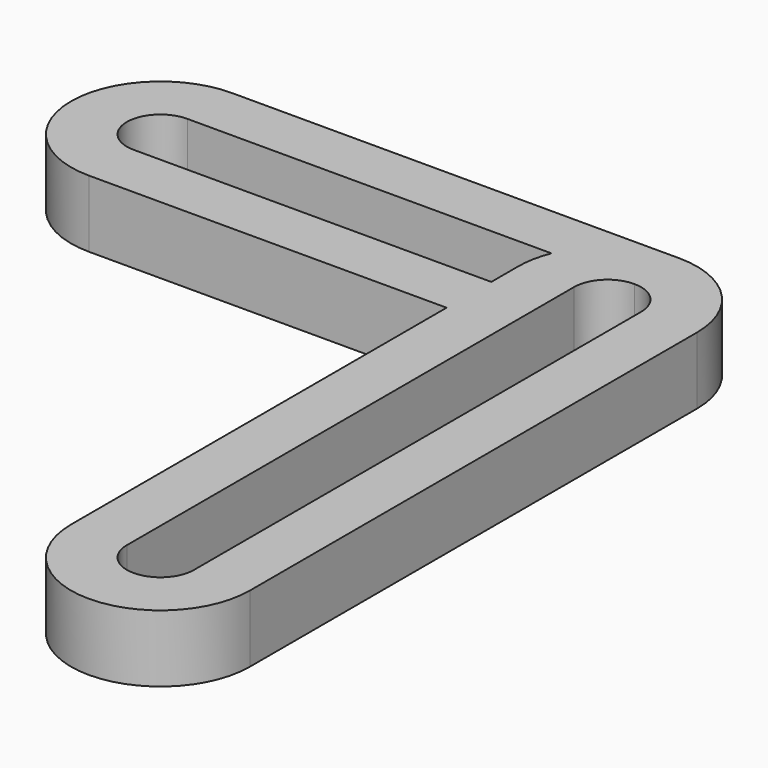
from build123d import *

# Parameters (mm, degrees)
F0_W     = 10
F0_H     = 10
F1_DEPTH = 12


# Not quite as in the source:
# - ends of sketch curves that miss each other by under 0.0002 mm in the source are joined


with BuildPart() as f1:
    # F0 (on Top) → F1 (new body)
    with BuildSketch(Plane.XY):
        with BuildLine():
            ThreePointArc((49.3437788486, 31.9918581452), (44.6574873088, 43.3055665732), (33.3437788486, 47.9918580353))
            ThreePointArc((33.3437788486, 47.9918580353), (24.3995068895, 45.2583572735), (18.51138183, 37.9918580353))
            Line((18.51138183, 37.9918580353), (33.3437788486, 37.9918580353))
            ThreePointArc((33.3437788486, 37.9918580353), (37.5864194969, 36.2344987613), (39.3437788486, 31.9918581452))
            Line((39.3437788486, 31.9918581452), (39.3437788486, 17.1594610611))
            ThreePointArc((39.3437788486, 17.1594610611), (46.6102780408, 23.0475861709), (49.3437788486, 31.9918581452))
        make_face()
        with BuildLine():
            Line((49.3437788486, -68.0081418548), (49.3437788486, 31.9918581452))
            ThreePointArc((49.3437788486, 31.9918581452), (46.6102780408, 23.0475861709), (39.3437788486, 17.1594610611))
            Line((39.3437788486, 17.1594610611), (39.3437788486, -68.0081418548))
            ThreePointArc((39.3437788486, -68.0081418548), (33.3437788486, -74.0081418548), (27.3437788486, -68.0081418548))
            Line((27.3437788486, -68.0081418548), (27.3437788486, 15.9918580353))
            Line((27.3437788486, 15.9918580353), (17.3437788486, 15.9918580353))
            Line((17.3437788486, 15.9918580353), (17.3437788486, -68.0081418548))
            ThreePointArc((17.3437788486, -68.0081418548), (33.3437788486, -84.0081418548), (49.3437788486, -68.0081418548))
        make_face()
        with BuildLine():
            Line((33.3437788486, 37.9918580353), (18.51138183, 37.9918580353))
            ThreePointArc((18.51138183, 37.9918580353), (17.6383919973, 35.0481342863), (17.3437788486, 31.9918581452))
            Line((17.3437788486, 31.9918581452), (17.3437788486, 25.9918580353))
            Line((17.3437788486, 25.9918580353), (27.3437788486, 25.9918580353))
            Line((27.3437788486, 25.9918580353), (27.3437788486, 31.9918581452))
            ThreePointArc((27.3437788486, 31.9918581452), (29.1011381615, 36.2344988323), (33.3437788486, 37.9918580353))
        make_face()
        with Locations((22.3437788486, 20.9918580353)):
            Rectangle(F0_W, F0_H)
        with BuildLine():
            Line((33.3437788486, 47.9918580353), (-46.6562211514, 47.9918580353))
            ThreePointArc((-46.6562211514, 47.9918580353), (-62.6562211514, 31.9918580353), (-46.6562211514, 15.9918580353))
            Line((-46.6562211514, 15.9918580353), (17.3437788486, 15.9918580353))
            Line((17.3437788486, 15.9918580353), (17.3437788486, 25.9918580353))
            Line((17.3437788486, 25.9918580353), (-46.6562211514, 25.9918580353))
            ThreePointArc((-46.6562211514, 25.9918580353), (-52.6562211514, 31.9918580353), (-46.6562211514, 37.9918580353))
            Line((-46.6562211514, 37.9918580353), (18.51138183, 37.9918580353))
            ThreePointArc((18.51138183, 37.9918580353), (24.3995068895, 45.2583572735), (33.3437788486, 47.9918580353))
        make_face()
    extrude(amount=F1_DEPTH)


solid = f1.part
